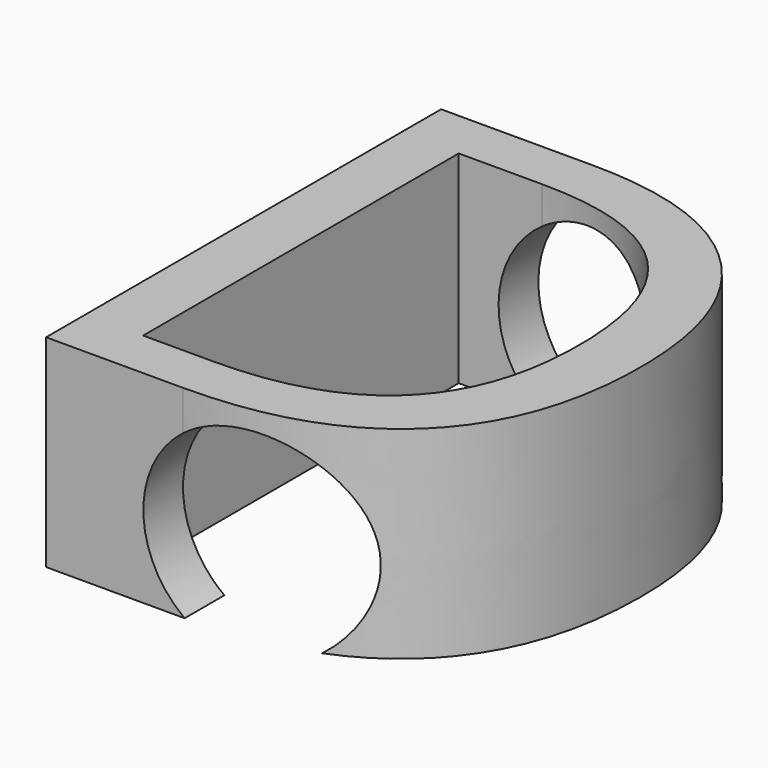
from build123d import *

# Parameters (mm, degrees)
F0_TEXT_SIZE = 85.4645390064
F1_DEPTH     = 25
F2_R         = 12.5679133389
F3_DEPTH     = 84.0540435165


# Not quite as in the source:
# - Text() gives the source's letters only with a copy of the font that has no kerning and outlines rounded to 1/6400 em; it was checked with that copy


with BuildPart() as f1:
    # F0 (on Top) → F1 (new body)
    with BuildSketch(Plane.XY):
        with Locations((-28.7748930035, 0)):
            Text('D', F0_TEXT_SIZE, font='Open Sans', text_align=(TextAlign.LEFT, TextAlign.BOTTOM))
    extrude(amount=F1_DEPTH)

    # F2 (on Front) → F3 (cut)
    with BuildSketch(Plane.XZ):
        with Locations((4.1973888874, 10.1095288992)):
            Circle(F2_R)
    extrude(amount=-F3_DEPTH, mode=Mode.SUBTRACT)


solid = f1.part
